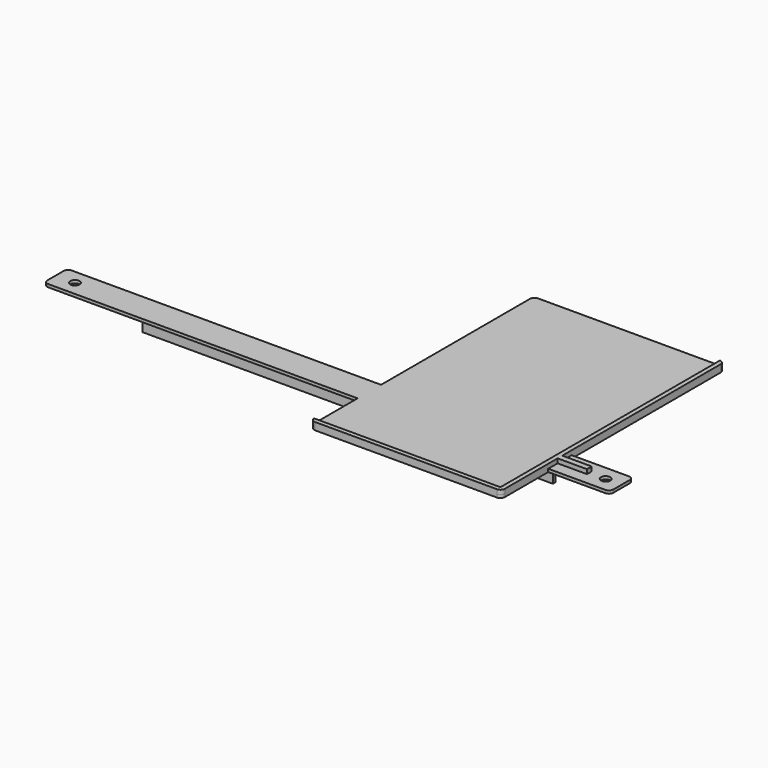
from build123d import *

# Parameters (mm, degrees)
F0_R     = 1.6
F1_DEPTH = 1
F2_R     = 1.5
F3_W     = 140
F3_H     = 1
F4_DEPTH = 6
F5_W     = 63.5
F5_H     = 1.5
F5_W_2   = 1.5
F5_H_2   = 93.5
F6_DEPTH = 1.5
F7_R     = 1.4999
F8_W     = 10
F8_H     = 2
F9_DEPTH = 1.5


# Not quite as in the source:
# - a fillet or chamfer is up to 0.001 mm smaller than in the source, because OpenCascade refuses the exact size


with BuildPart() as f1:
    # F0 (on Top) → F1 (new body)
    with BuildSketch(Plane.XY):
        Polygon((69.4188682817, 0), (-37.5811317183, 0), (-37.5811317183, -10), (69.4188682817, -10), (69.4188682817, -30), (134.4188682817, -30), (134.4188682817, -10), (155.4188682817, -10), (155.4188682817, 0), (134.4188682817, 0), (134.4188682817, 65), (69.4188682817, 65), align=None)
        with Locations((-30.9811317183, -5)):
            Circle(F0_R, mode=Mode.SUBTRACT)
        with Locations((150.0188682817, -5)):
            Circle(F0_R, mode=Mode.SUBTRACT)
    extrude(amount=F1_DEPTH)

    # F2
    f2_edges = [f1.edges().sort_by_distance(p)[0] for p in [
        (-37.581132, 0, 0.5),
        (-37.581132, -10, 0.5),
        (155.418868, 0, 0.5),
        (155.418868, -10, 0.5),
        (134.418868, -30, 0.5),
        (69.418868, -30, 0.5),
        (69.418868, 65, 0.5),
        (134.418868, 65, 0.5),
    ]]
    fillet(f2_edges, radius=F2_R)

    # F3 (on face) → F4 (join)
    with BuildSketch(Plane(origin=(0, 0, 0), x_dir=(1, 0, 0), z_dir=(0, 0, -1))):
        with Locations((62.4188682817, 5)):
            Rectangle(F3_W, F3_H)
    extrude(amount=F4_DEPTH)

    # F5 (on face) → F6 (join)
    with BuildSketch(Plane.XY.offset(1)):
        with Locations((101.1688682817, -29.25)):
            Rectangle(F5_W, F5_H)
        with Locations((133.6688682817, 18.25)):
            Rectangle(F5_W_2, F5_H_2)
        with Locations((133.6688682817, -29.25)):
            Rectangle(F5_W_2, F5_H)
    extrude(amount=F6_DEPTH)

    # F7 (radius 1.5 in the source; OpenCascade refuses exactly that, so slightly less here)
    f7_edges = [f1.edges().sort_by_distance(p)[0] for p in [
        (134.418868, -30, 1.75),
        (69.418868, -30, 1.75),
        (134.418868, 65, 1.75),
    ]]
    fillet(f7_edges, radius=F7_R)

    # F8 (on face) → F9 (join, through all)
    with BuildSketch(Plane.XY.offset(1)):
        with Locations((139.4188682817, -5)):
            Rectangle(F8_W, F8_H)
    extrude(amount=F9_DEPTH)


solid = f1.part
